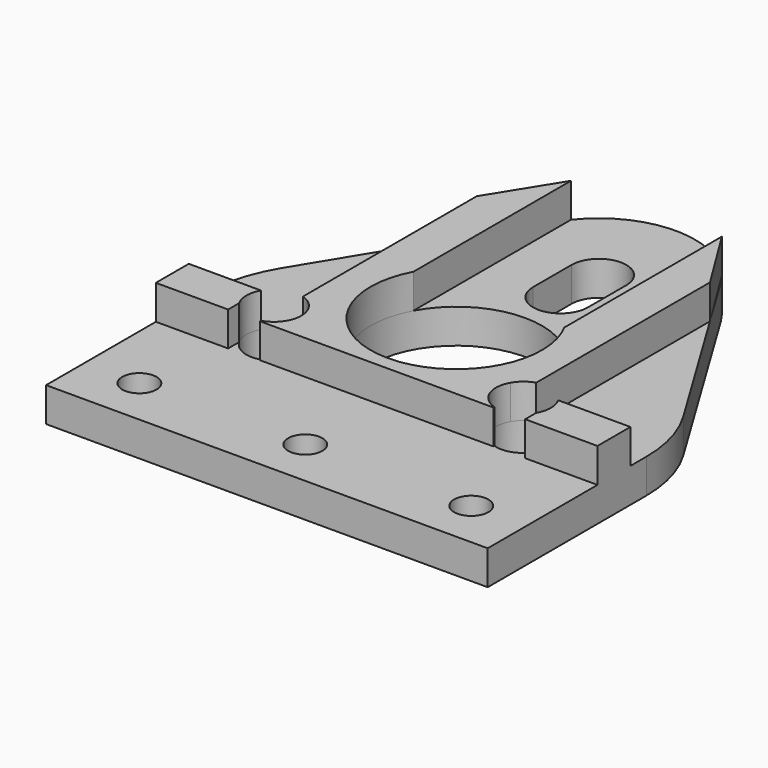
from build123d import *

# Parameters (mm, degrees)
F0_R     = 2.5
F0_R_2   = 4
F0_R_3   = 12.5
F1_DEPTH = 5
F3_DEPTH = 5


# Not quite as in the source:
# - after a boolean that leaves OpenCascade's solid faulty, fix() repairs it


with BuildPart() as f1:
    # F0 (on Top) → F1 (new body)
    with BuildSketch(Plane.XY):
        with BuildLine():
            Line((-32.1865334795, -5.601415029), (-32.1865334795, -34.5))
            Line((-32.1865334795, -34.5), (32.1865334795, -34.5))
            Line((32.1865334795, -34.5), (32.1865334795, -5.601415029))
            ThreePointArc((32.1865334795, -5.601415029), (31.4454600423, -0.2075529944), (29.2771587146, 4.7865842524))
            Line((29.2771587146, 4.7865842524), (11.9634376646, 33.271599497))
            ThreePointArc((11.9634376646, 33.271599497), (0, 40), (-11.9634376646, 33.271599497))
            Line((-11.9634376646, 33.271599497), (-29.2771587146, 4.7865842524))
            ThreePointArc((-29.2771587146, 4.7865842524), (-31.4454600423, -0.2075529944), (-32.1865334795, -5.601415029))
        make_face()
        with Locations((-24.1865334795, -27.5)):
            Circle(F0_R, mode=Mode.SUBTRACT)
        with Locations((-18.1865334795, -10.5)):
            Circle(F0_R_2, mode=Mode.SUBTRACT)
        with Locations((0, -27.5)):
            Circle(F0_R, mode=Mode.SUBTRACT)
        with Locations((24.1865334795, -27.5)):
            Circle(F0_R, mode=Mode.SUBTRACT)
        Circle(F0_R_3, mode=Mode.SUBTRACT)
        with Locations((18.1865334795, -10.5)):
            Circle(F0_R_2, mode=Mode.SUBTRACT)
        with BuildLine():
            Line((-4, 21), (-4, 26))
            ThreePointArc((-4, 26), (0, 30), (4, 26))
            Line((4, 26), (4, 21))
            Line((4, 21), (4, 19))
            ThreePointArc((4, 19), (0, 15), (-4, 19))
            Line((-4, 19), (-4, 21))
        make_face(mode=Mode.SUBTRACT)
    extrude(amount=F1_DEPTH)

    # F2 (on face) → F3 (join)
    with BuildSketch(Plane.XY.offset(5)):
        with BuildLine():
            Line((-32.1865334795, -8.5), (-32.1865334795, -14.5))
            Line((-32.1865334795, -14.5), (-21.6506350946, -14.5))
            Line((-21.6506350946, -14.5), (-21.6506350946, -12.5))
            ThreePointArc((-21.6506350946, -12.5), (-22.1865334795, -10.5), (-21.6506350946, -8.5))
            Line((-21.6506350946, -8.5), (-32.1865334795, -8.5))
        make_face()
        with BuildLine():
            Line((21.6506350946, -14.5), (32.1865334795, -14.5))
            Line((32.1865334795, -14.5), (32.1865334795, -8.5))
            Line((32.1865334795, -8.5), (21.6506350946, -8.5))
            ThreePointArc((21.6506350946, -8.5), (22.1865334795, -10.5), (21.6506350946, -12.5))
            Line((21.6506350946, -12.5), (21.6506350946, -14.5))
        make_face()
        with BuildLine():
            ThreePointArc((17, -14.3199657462), (14.4616036791, -11.9577029816), (14.7224318643, -8.5))
            ThreePointArc((14.7224318643, -8.5), (15.6895011358, -7.3751272866), (17, -6.6800342538))
            Line((17, -6.6800342538), (17, 24.9853071114))
            Line((17, 24.9853071114), (11, 34.6602540378))
            Line((11, 34.6602540378), (11, 5.9371710435))
            ThreePointArc((11, 5.9371710435), (0, -12.5), (-11, 5.9371710435))
            Line((-11, 5.9371710435), (-11, 34.6602540378))
            Line((-11, 34.6602540378), (-17, 24.9853071114))
            Line((-17, 24.9853071114), (-17, -6.6800342538))
            ThreePointArc((-17, -6.6800342538), (-15.6895011358, -7.3751272866), (-14.7224318643, -8.5))
            ThreePointArc((-14.7224318643, -8.5), (-14.4616036791, -11.9577029816), (-17, -14.3199657462))
            Line((-17, -14.3199657462), (-17, -14.5))
            Line((-17, -14.5), (17, -14.5))
            Line((17, -14.5), (17, -14.3199657462))
        make_face()
    extrude(amount=F3_DEPTH)

    add(f1.part.fix(), mode=Mode.REPLACE)


solid = f1.part
